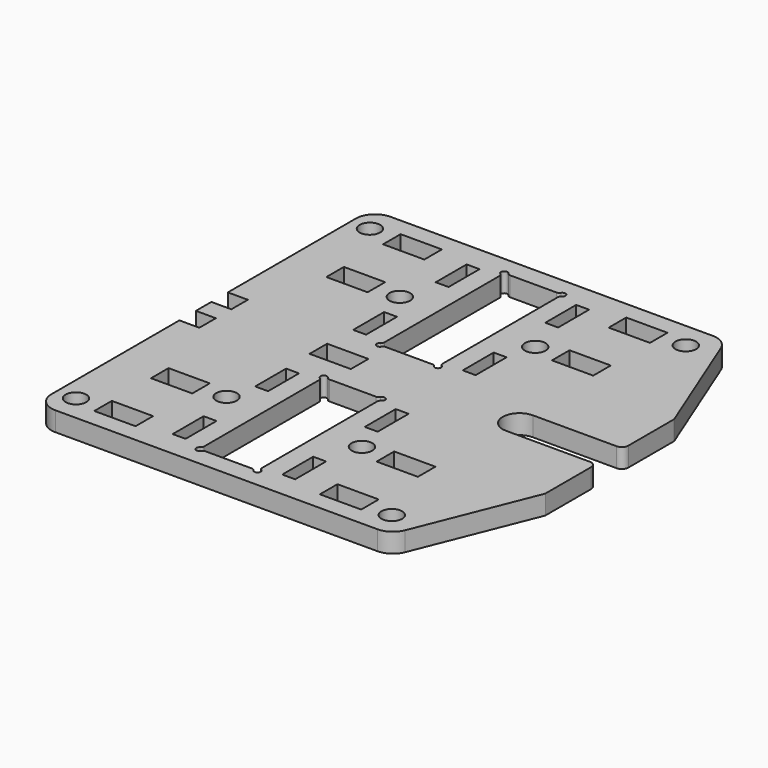
from build123d import *

# Parameters (mm, degrees)
F0_R     = 1.6
F0_W     = 6.4
F0_H     = 3.4
F0_W_2   = 2
F0_H_2   = 6
F1_DEPTH = 3


# Not quite as in the source:
# - ends of sketch curves that miss each other by under 0.0002 mm in the source are joined


with BuildPart() as f1:
    # F0 (on Top) → F1 (new body)
    with BuildSketch(Plane.XY):
        with BuildLine():
            Line((-31.5, 1.5), (-31.5, -1.5))
            Line((-31.5, -1.5), (-28.4, -1.5))
            Line((-28.4, -1.5), (-28.4, -4.7))
            Line((-28.4, -4.7), (-31.5, -4.7))
            Line((-31.5, -4.7), (-31.5, -29.5))
            ThreePointArc((-31.5, -29.5), (-30.6213203436, -31.6213203436), (-28.5, -32.5))
            Line((-28.5, -32.5), (21.468901, -32.5))
            ThreePointArc((21.468901, -32.5), (23.1507874279, -31.9842016914), (24.2543310727, -30.6141720291))
            Line((24.2543310727, -30.6141720291), (31.5, -12.5))
            Line((31.5, -12.5), (31.5, -3.6))
            ThreePointArc((31.5, -3.6), (31.2071067812, -2.8928932188), (30.5, -2.6))
            Line((30.5, -2.6), (17.5, -2.6))
            ThreePointArc((17.5, -2.6), (14.9, 0), (17.5, 2.6))
            Line((17.5, 2.6), (30.5, 2.6))
            ThreePointArc((30.5, 2.6), (31.2071067812, 2.8928932188), (31.5, 3.6))
            Line((31.5, 3.6), (31.5, 12.5))
            Line((31.5, 12.5), (24.2543, 30.6142))
            ThreePointArc((24.2543, 30.6142), (23.1507874279, 31.9842016914), (21.468901, 32.5))
            Line((21.468901, 32.5), (-28.5, 32.5))
            ThreePointArc((-28.5, 32.5), (-30.6213203436, 31.6213203436), (-31.5, 29.5))
            Line((-31.5, 29.5), (-31.5, 4.7))
            Line((-31.5, 4.7), (-28.4, 4.7))
            Line((-28.4, 4.7), (-28.4, 1.5))
            Line((-28.4, 1.5), (-31.5, 1.5))
        make_face()
        with Locations((-28.5, -28.5)):
            Circle(F0_R, mode=Mode.SUBTRACT)
        with Locations((-21.5, -28)):
            Rectangle(F0_W, F0_H, mode=Mode.SUBTRACT)
        with Locations((-21.5, -17)):
            Rectangle(F0_W, F0_H, mode=Mode.SUBTRACT)
        with Locations((-12.5, -25.5)):
            Rectangle(F0_W_2, F0_H_2, mode=Mode.SUBTRACT)
        with Locations((-14.5, -16.8)):
            Circle(F0_R, mode=Mode.SUBTRACT)
        with BuildLine():
            ThreePointArc((-8.0669872236, -29.8000098709), (-8.8535526014, -29.9035641797), (-8.7500018039, -29.1169983396))
            ThreePointArc((-8.7500018039, -29.1169983396), (-8.5669873354, -28.9339800645), (-8.5, -28.68398))
            Line((-8.5, -28.68398), (-8.5, -6.316))
            ThreePointArc((-8.5, -6.316), (-8.5669873354, -6.0659999355), (-8.7500001291, -5.8829872236))
            ThreePointArc((-8.7500001291, -5.8829872236), (-8.8535533906, -5.0964466094), (-8.0669872236, -5.2000001291))
            ThreePointArc((-8.0669872236, -5.2000001291), (-7.8840000645, -5.3830126646), (-7.634, -5.45))
            Line((-7.634, -5.45), (-0.366, -5.45))
            ThreePointArc((-0.366, -5.45), (-0.1159999355, -5.3830126646), (0.0670127764, -5.1999998709))
            ThreePointArc((0.0670127764, -5.1999998709), (0.8535541797, -5.0964473986), (0.7499998709, -5.8830127764))
            ThreePointArc((0.7499998709, -5.8830127764), (0.5669873354, -6.0659999355), (0.5, -6.316))
            Line((0.5, -6.316), (0.5, -28.68397))
            ThreePointArc((0.5, -28.68397), (0.5669873354, -28.9339700645), (0.7500001291, -29.1169827764))
            ThreePointArc((0.7500001291, -29.1169827764), (0.8535533906, -29.9035533906), (0.0669872236, -29.7999998709))
            ThreePointArc((0.0669872236, -29.7999998709), (-0.1159999355, -29.6169873354), (-0.366, -29.55))
            Line((-0.366, -29.55), (-7.634, -29.55001))
            ThreePointArc((-7.634, -29.55001), (-7.8840000645, -29.6169973354), (-8.0669872236, -29.8000098709))
        make_face(mode=Mode.SUBTRACT)
        with Locations((-12.5, -9.5)):
            Rectangle(F0_W_2, F0_H_2, mode=Mode.SUBTRACT)
        with Locations((4.5, -25.5)):
            Rectangle(F0_W_2, F0_H_2, mode=Mode.SUBTRACT)
        with Locations((13.5, -28)):
            Rectangle(F0_W, F0_H, mode=Mode.SUBTRACT)
        with Locations((6.5, -16.8)):
            Circle(F0_R, mode=Mode.SUBTRACT)
        with Locations((13.5, -17)):
            Rectangle(F0_W, F0_H, mode=Mode.SUBTRACT)
        with Locations((20.5, -28.5)):
            Circle(F0_R, mode=Mode.SUBTRACT)
        with Locations((4.5, -9.5)):
            Rectangle(F0_W_2, F0_H_2, mode=Mode.SUBTRACT)
        with Locations((-10.5, 0)):
            Rectangle(F0_W, F0_H, mode=Mode.SUBTRACT)
        with Locations((-12.5, 9.5)):
            Rectangle(F0_W_2, F0_H_2, mode=Mode.SUBTRACT)
        with Locations((-21.5, 17)):
            Rectangle(F0_W, F0_H, mode=Mode.SUBTRACT)
        with Locations((-28.5, 28.5)):
            Circle(F0_R, mode=Mode.SUBTRACT)
        with Locations((-21.5, 28)):
            Rectangle(F0_W, F0_H, mode=Mode.SUBTRACT)
        with Locations((-14.5, 16.8)):
            Circle(F0_R, mode=Mode.SUBTRACT)
        with BuildLine():
            ThreePointArc((-8.0669772236, 5.1999911291), (-8.8535424247, 5.0964366435), (-8.7499922369, 5.8830024104))
            ThreePointArc((-8.7499922369, 5.8830024104), (-8.5669772104, 6.066020152), (-8.49999, 6.31602))
            Line((-8.49999, 6.31602), (-8.49999, 28.684))
            ThreePointArc((-8.49999, 28.684), (-8.5669773354, 28.9340000645), (-8.7499901291, 29.1170127764))
            ThreePointArc((-8.7499901291, 29.1170127764), (-8.8535432138, 29.9035535674), (-8.0669772236, 29.7999998709))
            ThreePointArc((-8.0669772236, 29.7999998709), (-7.8839900645, 29.6169873354), (-7.63399, 29.55))
            Line((-7.63399, 29.55), (-0.36599, 29.55))
            ThreePointArc((-0.36599, 29.55), (-0.1159899355, 29.6169873354), (0.0670227764, 29.8000001291))
            ThreePointArc((0.0670227764, 29.8000001291), (0.853564003, 29.9035527782), (0.7500103039, 29.1169874736))
            ThreePointArc((0.7500103039, 29.1169874736), (0.5669973354, 28.9340000645), (0.50001, 28.684))
            Line((0.50001, 28.684), (0.50001, 6.316031))
            ThreePointArc((0.50001, 6.316031), (0.5669973354, 6.0660309355), (0.7500101291, 5.8830182236))
            ThreePointArc((0.7500101291, 5.8830182236), (0.8535633906, 5.0964466094), (0.0669972236, 5.2000001291))
            ThreePointArc((0.0669972236, 5.2000001291), (-0.1159899355, 5.3830126646), (-0.36599, 5.45))
            Line((-0.36599, 5.45), (-7.63399, 5.449991))
            ThreePointArc((-7.63399, 5.449991), (-7.8839900645, 5.3830036646), (-8.0669772236, 5.1999911291))
        make_face(mode=Mode.SUBTRACT)
        with Locations((-12.5, 25.5)):
            Rectangle(F0_W_2, F0_H_2, mode=Mode.SUBTRACT)
        with Locations((4.5, 9.5)):
            Rectangle(F0_W_2, F0_H_2, mode=Mode.SUBTRACT)
        with Locations((6.5, 16.8)):
            Circle(F0_R, mode=Mode.SUBTRACT)
        with Locations((13.5, 17)):
            Rectangle(F0_W, F0_H, mode=Mode.SUBTRACT)
        with Locations((4.5, 25.5)):
            Rectangle(F0_W_2, F0_H_2, mode=Mode.SUBTRACT)
        with Locations((13.5, 28)):
            Rectangle(F0_W, F0_H, mode=Mode.SUBTRACT)
        with Locations((20.5, 28.5)):
            Circle(F0_R, mode=Mode.SUBTRACT)
    extrude(amount=F1_DEPTH)


solid = f1.part
